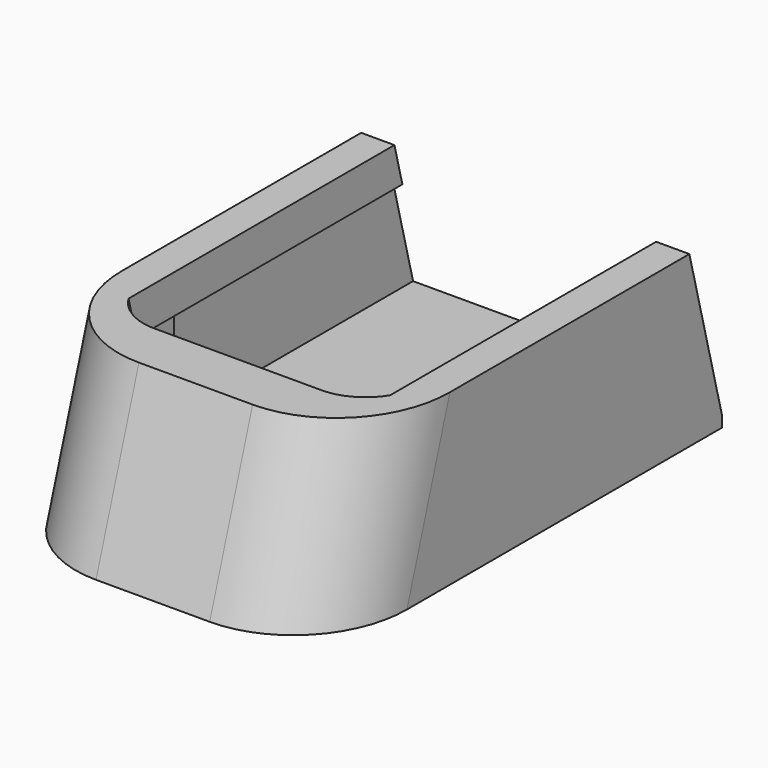
from build123d import *

# Parameters (mm, degrees)
F3_DEPTH    = 13
F4_DEPTH    = 12.2
F5_T1_DEPTH = 35.5
F6_DEPTH    = 15.3
F7_R        = 10
F8_DEPTH    = 28.5
F10_R       = 1.85
F11_DEPTH   = 5
F14_DEPTH   = 20


# Not quite as in the source:
# - a fillet or chamfer that OpenCascade refuses, or shapes differently, is made with other operations: its cross-section is extruded or revolved along the edge and cut away or added


with BuildPart() as f3:
    # F2 (on Right) → F3 (new body, symmetric)
    with BuildSketch(Plane.YZ):
        Polygon((-5.5, 3), (0, 3), (28, 3), (25.6314561435, 12.2), (-7.8685438565, 12.2), align=None)
    extrude(amount=F3_DEPTH, both=True)

    # F2 (on Right) → F4 (join, symmetric)
    with BuildSketch(Plane.YZ):
        Polygon((-8.7953653655, 15.8), (-7.8685438565, 12.2), (25.6314561435, 12.2), (24.7046346345, 15.8), align=None)
    extrude(amount=F4_DEPTH, both=True)

    # F5: fillet of radius 5.2 on 2 edges, made by hand

    # F5_s2 → F5_t1 (cut)
    with BuildSketch(Plane(origin=(0, -6.6759341801, 25.9309509046), x_dir=(1, 0, 0), z_dir=(0, 0.2493204059, -0.9684210526))):
        with BuildLine():
            ThreePointArc((7.8, 4.5783545716), (11.4769552622, 3.0553098338), (13, -0.6216454284))
            Line((13, -0.6216454284), (13, 4.5783545716))
            Line((13, 4.5783545716), (7.8, 4.5783545716))
        make_face()
        with BuildLine():
            ThreePointArc((-7.8, 4.5783545716), (-11.4769552622, 3.0553098338), (-13, -0.6216454284))
            Line((-13, -0.6216454284), (-13, 4.5783545716))
            Line((-13, 4.5783545716), (-7.8, 4.5783545716))
        make_face()
    extrude(amount=F5_T1_DEPTH, mode=Mode.SUBTRACT)


with BuildPart() as f6:
    # F1 (on Right) → F6 (new body, symmetric)
    with BuildSketch(Plane.YZ):
        Polygon((-18.7, 0), (0, 0), (0, 15.8), (-13.7, 15.8), align=None)
    extrude(amount=F6_DEPTH, both=True)

    # F7
    f7_edges = [f6.edges().sort_by_distance(p)[0] for p in [
        (15.3, -16.2, 7.9),
        (-15.3, -16.2, 7.9),
    ]]
    fillet(f7_edges, radius=F7_R)

    # F0 (on Front) → F8 (join)
    with BuildSketch(Plane.XZ):
        Polygon((-15.3, 0), (0, 0), (15.3, 0), (15.3, 15.8), (12.2, 15.8), (12.2, 12.2), (13.1, 12.2), (13.1, 3), (0, 3), (-13.1, 3), (-13.1, 12.2), (-12.2, 12.2), (-12.2, 15.8), (-15.3, 15.8), align=None)
    extrude(amount=-F8_DEPTH)

    # F9: cut F3
    add(f3.part, mode=Mode.SUBTRACT)


with BuildPart() as f11:
    # F10 (on Top) → F11 (new body)
    with BuildSketch(Plane.XY):
        Circle(F10_R)
    extrude(amount=F11_DEPTH)


with BuildPart() as f6_1:
    add(f6.part)

    # F12: cut F11
    add(f11.part, mode=Mode.SUBTRACT)

    # F13 (on Right) → F14 (cut, symmetric)
    with BuildSketch(Plane.YZ):
        Polygon((29.3071324871, 15.8), (24.7046346345, 15.8), (28, 3), (29.3071324871, -2.0772202713), align=None)
    extrude(amount=F14_DEPTH, both=True, mode=Mode.SUBTRACT)


solid = f6_1.part
